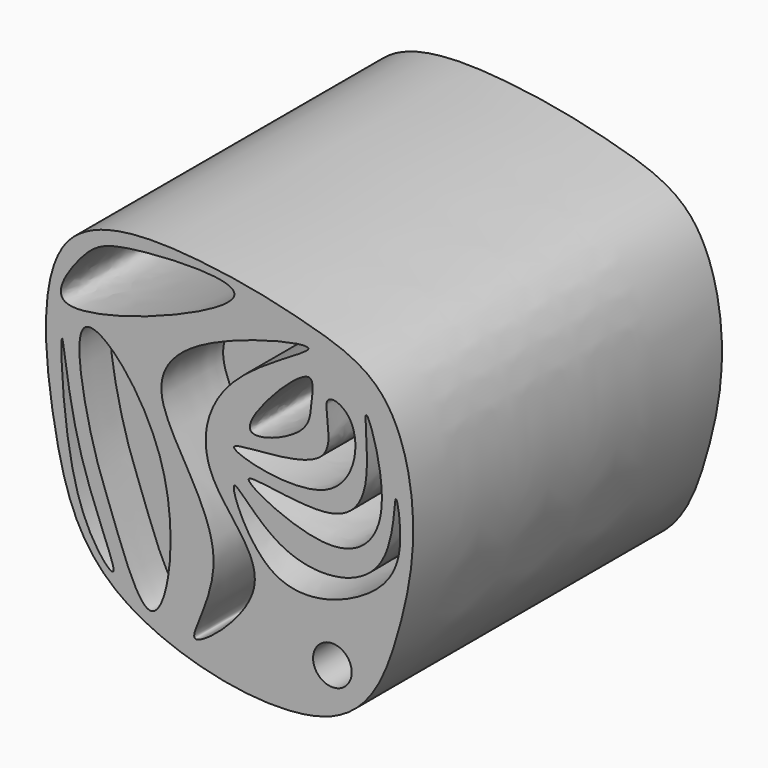
from build123d import *

# Parameters (mm, degrees)
F2_DEPTH  = 25.4
F4_DEPTH  = 25.4
F6_D      = 2.54
F8_DEPTH  = 2.54
F10_DEPTH = 5.08
F12_DEPTH = 2.54


with BuildPart() as f2:
    # F1 (on face) → F2 (new body)
    with BuildSketch(Plane.XZ):
        with BuildLine():
            add(Edge.make_bspline(
                [(-19.5936542004, 18.2083770633), (-17.7989219876, 20.227046702), (-10.6844767591, 20.111268629), (-3.9762354129, 18.6279469735), (1.7787329985, 16.7719928214), (3.6190010529, 9.3130036563), (2.2843808579, 2.4633033198), (-0.9486224503, -6.0711815231), (-17.6434316729, -2.8559570949), (-20.8108767682, 6.3101505118), (-21.6347675564, 15.9125841137), (-19.5936542004, 18.2083770633)],
                knots=[0, 0, 0, 0, 0.1127815622, 0.2166544922, 0.3049007165, 0.4045808789, 0.5074484566, 0.6112822946, 0.7529144332, 0.8717357658, 1, 1, 1, 1], degree=3))
        make_face()
    extrude(amount=F2_DEPTH)

    # F3 (on face) → F4 (cut)
    with BuildSketch(Plane.XZ.offset(25.4)):
        with BuildLine():
            add(Edge.make_bspline(
                [(-18.8149716705, 17.4296926707), (-17.918360896, 18.4778018007), (-16.4072310705, 19.2839890325), (-2.3075885354, 19.8087139609), (-22.6090250496, 12.0160473192), (-19.6178418597, 16.491163267), (-18.8149716705, 17.4296926707)],
                knots=[0, 0, 0, 0, 0.19964111, 0.4677325262, 0.8212313522, 1, 1, 1, 1], degree=3))
        make_face()
        with BuildLine():
            add(Edge.make_bspline(
                [(-20.0262572616, 12.4115087092), (-20.1382573386, 12.1341375663), (-19.9122362065, 3.0224567635), (-15.2527453645, -1.8885484621), (-19.4050822571, 5.8947899146), (-19.9341150995, 12.6397012025), (-20.0262572616, 12.4115087092)],
                knots=[0, 0, 0, 0, 0.3013578893, 0.4969267166, 0.752073675, 1, 1, 1, 1], degree=3))
        make_face()
        with BuildLine():
            add(Edge.make_bspline(
                [(-3.8469396532, 15.4397236183), (-4.7224321363, 15.3672950619), (-10.2474224349, 9.5468290111), (-3.675909362, 11.9217759182), (-3.6615249721, 13.827050084), (-3.4249915402, 15.4746309343), (-3.8469396532, 15.4397236183)],
                knots=[0, 0, 0, 0, 0.3480475526, 0.6135672143, 0.8322566888, 1, 1, 1, 1], degree=3))
        make_face()
        with BuildLine():
            add(Edge.make_bspline(
                [(-2.5491337292, 14.4879985601), (-2.8780825167, 13.9717314706), (-0.8203898338, 9.7085789362), (-12.941534472, 10.4992873672), (-1.1413514516, 7.3527183071), (-0.1001726568, 14.1075256971), (-2.3209581175, 14.8461076743), (-2.5491337292, 14.4879985601)],
                knots=[0, 0, 0, 0, 0.1784873606, 0.4181378506, 0.6601644277, 0.8761920876, 1, 1, 1, 1], degree=3))
        make_face()
        with BuildLine():
            add(Edge.make_bspline(
                [(0, 14.4879985601), (-0.1824724002, 14.4889138687), (0.5360897106, 10.2725565194), (-1.7606304417, 7.0075757881), (-10.8727567866, 9.48579364), (-1.897654201, 4.7540053355), (2.151472136, 8.6490982831), (0.2183095876, 14.4869034868), (0, 14.4879985601)],
                knots=[0, 0, 0, 0, 0.14693372, 0.297732469, 0.4734615256, 0.6557196875, 0.8242088131, 1, 1, 1, 1], degree=3))
        make_face()
        with BuildLine():
            add(Edge.make_bspline(
                [(1.9499284681, 10.2484989911), (1.8126056723, 10.187993905), (2.0396913617, 4.5992089174), (-5.6296770796, 3.6178631481), (-9.8799367059, 9.834018916), (-6.6354019303, 1.394728179), (0.4753794053, 3.6965936669), (2.6479742963, 6.9199975506), (2.0599632715, 10.2969808562), (1.9499284681, 10.2484989911)],
                knots=[0, 0, 0, 0, 0.1367584681, 0.3069604939, 0.4415920238, 0.588638246, 0.7551484699, 0.8904173843, 1, 1, 1, 1], degree=3))
        make_face()
    extrude(amount=-F4_DEPTH, mode=Mode.SUBTRACT)

    # F6 (through all)
    with Locations(Plane(origin=(0, 0, 0), x_dir=(1, 0, 0), z_dir=(0, 1, 0))):
        with Locations((-2.228774596, 0.7417942397)):
            Hole(F6_D / 2)

    # F7 (on face) → F8 (cut)
    with BuildSketch(Plane.XZ.offset(25.4)):
        with BuildLine():
            add(Edge.make_bspline(
                [(-18.4875559062, 13.5579742491), (-19.3154822408, 12.9848281708), (-18.0697050928, 6.6511359386), (-16.9799538782, 4.1954561535), (-13.7433502687, -5.2416502841), (-11.4915391718, 7.7972606227), (-17.5311324309, 14.2200746573), (-18.4875559062, 13.5579742491)],
                knots=[0, 0, 0, 0, 0.193983347, 0.3582842909, 0.5429808015, 0.7759097408, 1, 1, 1, 1], degree=3))
        make_face()
    extrude(amount=-F8_DEPTH, mode=Mode.SUBTRACT)

    # F9 (on face) → F10 (cut)
    with BuildSketch(Plane.XZ.offset(25.4)):
        with BuildLine():
            add(Edge.make_bspline(
                [(-3.813148709, 17.107822001), (-3.6859754444, 16.809173885), (-10.0359252297, 14.0086392851), (-11.5248229669, 7.3300771967), (-4.7496793502, 2.6052117682), (-13.4784097518, -4.545289679), (-7.8127471121, 3.6130816702), (-15.3196319816, 11.1291138173), (-11.1589079567, 15.7046122726), (-3.9484000723, 17.4254403695), (-3.813148709, 17.107822001)],
                knots=[0, 0, 0, 0, 0.1226578002, 0.2469274469, 0.3721565583, 0.4920317284, 0.6042342176, 0.7554833356, 0.8695509253, 1, 1, 1, 1], degree=3))
        make_face()
    extrude(amount=-F10_DEPTH, mode=Mode.SUBTRACT)

    # F11 (on face) → F12 (join)
    with BuildSketch(Plane.XZ):
        with BuildLine():
            add(Edge.make_bspline(
                [(-7.5533334166, 16.0078406334), (-9.6134745729, 15.5015447096), (-12.939547657, 15.0528311828), (-18.5589879203, 14.2233845171), (-18.7383844377, 7.9567087911), (-15.5469458631, 1.2369371191), (-10.0917759326, -3.7645611405), (-1.9947567807, 0.1309326934), (-10.1031345222, 3.5347732827), (-10.4824045873, 10.4919778205), (-7.4844304912, 14.1528648853), (-2.2335307907, 17.56169165), (-5.9152217774, 16.4104194776), (-7.5533334166, 16.0078406334)],
                knots=[0, 0, 0, 0, 0.0942118734, 0.1789337345, 0.2673375082, 0.3759387605, 0.4788723113, 0.5684768295, 0.6629971261, 0.7602378038, 0.8495687287, 0.9250878679, 1, 1, 1, 1], degree=3))
        make_face()
    extrude(amount=F12_DEPTH)


solid = f2.part
